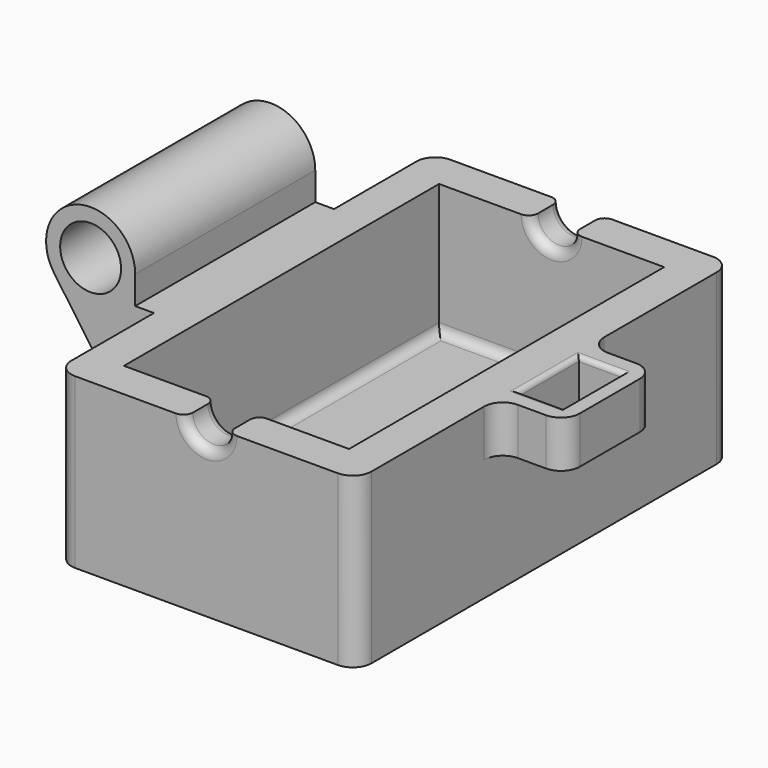
from build123d import *

# Parameters (mm, degrees)
F0_W          = 16
F0_H          = 25
F1_DEPTH      = 9
F2_T          = -2
F4_DEPTH      = 6
F5_R          = 1.625
F6_DEPTH      = 25
F7_R          = 1.125
F8_DEPTH      = 25
F8_DEPTH_BACK = 25
F9_R          = 1
F11_W         = 3.5
F11_H         = 6
F11_W_2       = 2
F11_H_2       = 4
F12_DEPTH     = 2.5
F13_R         = 1
F14_R         = 0.25
F15_SIZE2     = 1.3737387097
F15_SIZE      = 0.5
F16_R         = 0.5
F17_R         = 0.5


# Not quite as in the source:
# - two fillets or chamfers of one size are made in one step


with BuildPart() as f1:
    # F0 (on Top) → F1 (new body)
    with BuildSketch(Plane.XY):
        Rectangle(F0_W, F0_H)
    extrude(amount=-F1_DEPTH)

    # F2
    f2_openings = [f1.faces().sort_by_distance(p)[0] for p in [
        (0, 0, 0),
    ]]
    offset(amount=F2_T, openings=f2_openings)

    # F3 (on Front) → F4 (join, symmetric)
    with BuildSketch(Plane.XZ):
        with BuildLine():
            ThreePointArc((-9, 1.5), (-12.0919927986, 3.7641877852), (-13.3170916435, 0.1329209796))
            Line((-13.3170916435, 0.1329209796), (-9, -6))
            Line((-9, -6), (-8, -6))
            Line((-8, -6), (-8, 0))
            Line((-8, 0), (-9, 0))
            Line((-9, 0), (-9, 1.5))
        make_face()
    extrude(amount=F4_DEPTH, both=True)

    # F5 (on face) → F6 (cut)
    with BuildSketch(Plane(origin=(0, 6, 0), x_dir=(-1, 0, 0), z_dir=(0, 1, 0))):
        with Locations((11.375, 1.5)):
            Circle(F5_R)
    extrude(amount=-F6_DEPTH, mode=Mode.SUBTRACT)

    # F7 (on Front) → F8 (cut, two sides)
    with BuildSketch(Plane.XZ) as f8_sk:
        Circle(F7_R)
    extrude(amount=-F8_DEPTH, mode=Mode.SUBTRACT)
    extrude(f8_sk.sketch, amount=F8_DEPTH_BACK, mode=Mode.SUBTRACT)

    # F9
    f9_edges = [f1.edges().sort_by_distance(p)[0] for p in [
        (8, -12.5, -4.5),
        (8, 12.5, -4.5),
        (-8, -12.5, -4.5),
        (-8, 12.5, -4.5),
        (-9, 0, -6),
    ]]
    fillet(f9_edges, radius=F9_R)

    # F11 (on face) → F12 (join)
    with BuildSketch(Plane.XY):
        with Locations((9.75, 0)):
            Rectangle(F11_W, F11_H)
        with Locations((9.25, 0)):
            Rectangle(F11_W_2, F11_H_2, mode=Mode.SUBTRACT)
    extrude(amount=-F12_DEPTH)

    # F13
    f13_edges = [f1.edges().sort_by_distance(p)[0] for p in [
        (11.5, -3, -1.25),
        (8, -3, -1.25),
        (11.5, 3, -1.25),
        (8, 3, -1.25),
    ]]
    fillet(f13_edges, radius=F13_R)

    # F14
    f14_edges = [f1.edges().sort_by_distance(p)[0] for p in [
        (9.25, 2, 0),
        (8.25, 0, 0),
        (9.25, -2, 0),
    ]]
    fillet(f14_edges, radius=F14_R)

    # F15
    f15_edges = [f1.edges().sort_by_distance(p)[0] for p in [
        (10.25, 0, 0),
    ]]
    f15_side = f1.faces().sort_by_distance((6.594217, 0, 0))[0]
    chamfer(f15_edges, length=F15_SIZE, length2=F15_SIZE2, reference=f15_side)

    # F16
    f16_edges = [f1.edges().sort_by_distance(p)[0] for p in [
        (0, 12.5, -1.125),
        (0, -12.5, -1.125),
    ]]
    fillet(f16_edges, radius=F16_R)

    # F17
    f17_edges = [f1.edges().sort_by_distance(p)[0] for p in [
        (0, 10.5, -1.125),
        (0, 10.5, -7),
        (0, -10.5, -7),
        (6, 0, -7),
        (0, -10.5, -1.125),
        (-6, 0, -7),
    ]]
    fillet(f17_edges, radius=F17_R)


solid = f1.part
